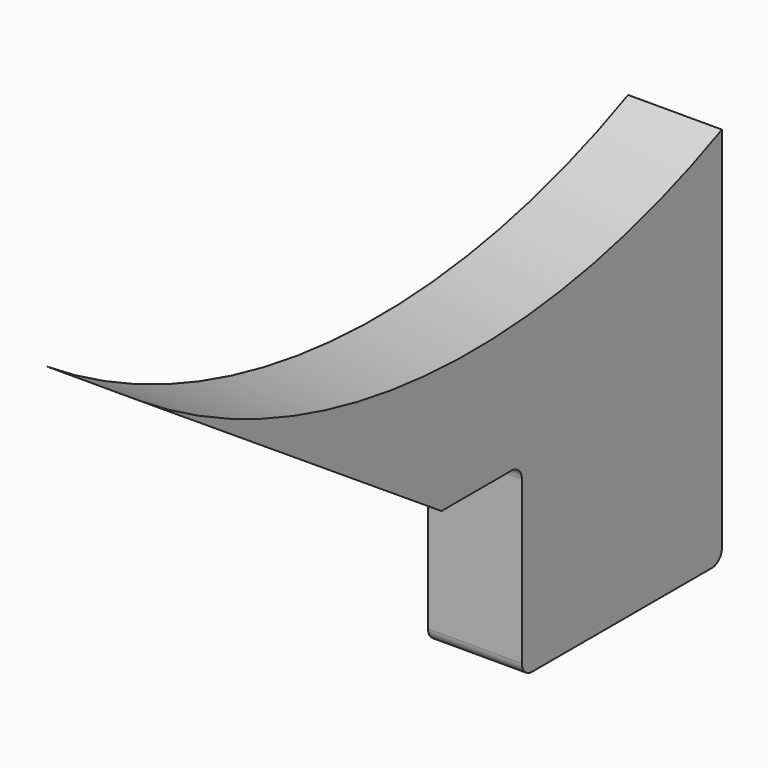
from build123d import *

# Parameters (mm, degrees)
F1_DEPTH = 0.75


# Not quite as in the source:
# - a feature names something its author has since deleted; it is built from what else it names


with BuildPart() as f1:
    # F0 (on Right) → F1 (new body, symmetric)
    with BuildSketch(Plane.YZ):
        with BuildLine():
            Line((-22.3, -0.8), (-22.3, 5.0912878854))
            ThreePointArc((-22.3, 5.0912878854), (-28.2361690228, 4.0365729174), (-33.9360169573, 6.0018362214))
            Line((-33.9360169573, 6.0018362214), (-27.9066450894, 2))
            Line((-27.9066450894, 2), (-26.5, 2))
            ThreePointArc((-26.5, 2), (-26.3585786438, 1.9414213562), (-26.3, 1.8))
            Line((-26.3, 1.8), (-26.3, -0.8))
            ThreePointArc((-26.3, -0.8), (-26.2414213562, -0.9414213562), (-26.1, -1))
            Line((-26.1, -1), (-22.5, -1))
            ThreePointArc((-22.5, -1), (-22.3585786438, -0.9414213562), (-22.3, -0.8))
        make_face()
    extrude(amount=F1_DEPTH, both=True)


solid = f1.part
